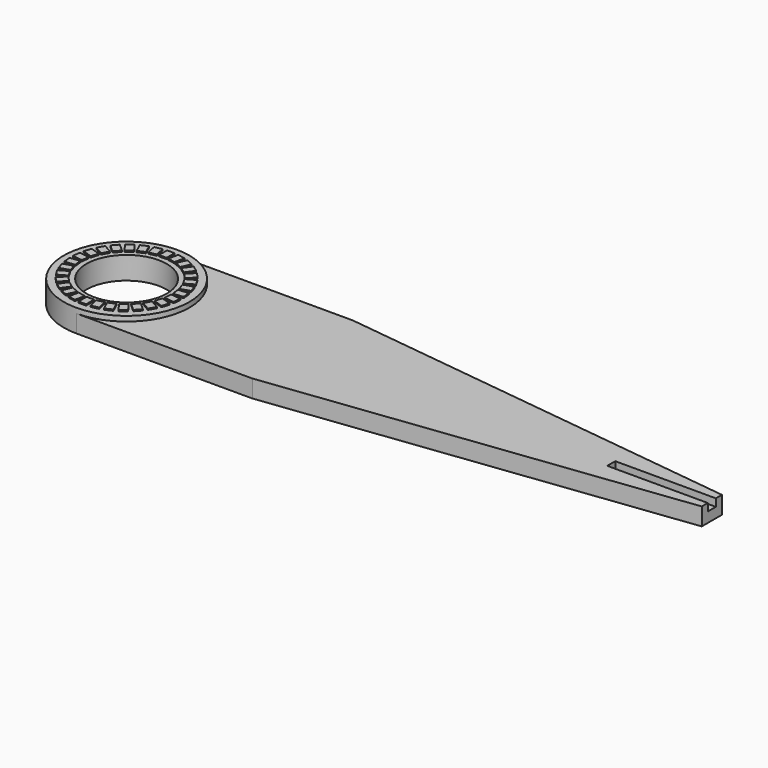
from build123d import *

# Parameters (mm, degrees)
F0_R         = 8
F1_DEPTH     = 3.5
F2_R         = 12.5
F2_R_2       = 8
F3_DEPTH     = 1
F4_W         = 1.5
F4_H         = 2
F5_DEPTH     = 0.25
F6_W         = 24.5562216001
F6_H         = 2
F6_W_2       = 20
F7_DEPTH     = 1.5
F9_TEXT_SIZE = 21.8350861027
F10_DEPTH    = 1.5


# Not quite as in the source:
# - Text() gives the source's letters only with a copy of the font that has no kerning and outlines rounded to 1/6400 em; it was checked with that copy


with BuildPart() as f1:
    # F0 (on Top) → F1 (new body)
    with BuildSketch(Plane.XY):
        with BuildLine():
            Line((35, 12.5), (0, 12.5))
            ThreePointArc((0, 12.5), (-12.5, 0), (0, -12.5))
            Line((0, -12.5), (35, -12.5))
            Line((35, -12.5), (116.3887844346, -2.5067138408))
            Line((116.3887844346, -2.5067138408), (116.3887844346, 2.5067138408))
            Line((116.3887844346, 2.5067138408), (35, 12.5))
        make_face()
        Circle(F0_R, mode=Mode.SUBTRACT)
    extrude(amount=F1_DEPTH)

    # F2 (on face) → F3 (join)
    with BuildSketch(Plane.XY.offset(3.5)):
        Circle(F2_R)
        Circle(F2_R_2, mode=Mode.SUBTRACT)
    extrude(amount=F3_DEPTH)

    # F4 (on face) → F5 (join)
    with BuildSketch(Plane.XY.offset(4.5)):
        with Locations((0, 10)):
            Rectangle(F4_W, F4_H)
        Polygon((-1.5534178984, 10.9155573762), (-3.0206392995, 10.60368984), (-2.6048159179, 8.6473946385), (-1.1375945168, 8.9592621747), align=None)
        Polygon((-3.7889439806, 10.3540525164), (-5.1592621671, 9.7439475518), (-4.3457888809, 7.9168566365), (-2.9754706945, 8.5269616011), align=None)
        Polygon((-5.8588750294, 9.3400258773), (-7.072400521, 8.4583479989), (-5.8968300164, 6.8403140102), (-4.6833045249, 7.7219918886), align=None)
        Polygon((-7.6727451255, 7.9177952891), (-8.676441035, 6.8030780508), (-7.1901513841, 5.4648168381), (-6.1864554745, 6.5795340763), align=None)
        Polygon((-9.1512794416, 6.1495190528), (-9.9012794416, 4.8504809472), (-8.1692286341, 3.8504809472), (-7.4192286341, 5.1495190528), align=None)
        Polygon((-10.2298589335, 4.1124793253), (-10.693384425, 2.6858945509), (-8.7912713924, 2.0678605622), (-8.3277459009, 3.4944453366), align=None)
        Polygon((-10.8613445016, 1.8957045175), (-11.0181371965, 0.4039216744), (-9.0290934058, 0.1948647479), (-8.8723007109, 1.6866475909), align=None)
        Polygon((-11.0181371965, -0.4039216744), (-10.8613445016, -1.8957045175), (-8.8723007109, -1.6866475909), (-9.0290934058, -0.1948647479), align=None)
        Polygon((-10.693384425, -2.6858945509), (-10.2298589335, -4.1124793253), (-8.3277459009, -3.4944453366), (-8.7912713924, -2.0678605622), align=None)
        Polygon((-9.9012794416, -4.8504809472), (-9.1512794416, -6.1495190528), (-7.4192286341, -5.1495190528), (-8.1692286341, -3.8504809472), align=None)
        Polygon((-8.676441035, -6.8030780508), (-7.6727451255, -7.9177952891), (-6.1864554745, -6.5795340763), (-7.1901513841, -5.4648168381), align=None)
        Polygon((-7.072400521, -8.4583479989), (-5.8588750294, -9.3400258773), (-4.6833045249, -7.7219918886), (-5.8968300164, -6.8403140102), align=None)
        Polygon((-5.1592621671, -9.7439475518), (-3.7889439806, -10.3540525164), (-2.9754706945, -8.5269616011), (-4.3457888809, -7.9168566365), align=None)
        Polygon((-3.0206392995, -10.60368984), (-1.5534178984, -10.9155573762), (-1.1375945168, -8.9592621747), (-2.6048159179, -8.6473946385), align=None)
        with Locations((0, -10)):
            Rectangle(F4_W, F4_H)
        Polygon((1.5534178984, -10.9155573762), (3.0206392995, -10.60368984), (2.6048159179, -8.6473946385), (1.1375945168, -8.9592621747), align=None)
        Polygon((3.7889439806, -10.3540525164), (5.1592621671, -9.7439475518), (4.3457888809, -7.9168566365), (2.9754706945, -8.5269616011), align=None)
        Polygon((5.8588750294, -9.3400258773), (7.072400521, -8.4583479989), (5.8968300164, -6.8403140102), (4.6833045249, -7.7219918886), align=None)
        Polygon((7.6727451255, -7.9177952891), (8.676441035, -6.8030780508), (7.1901513841, -5.4648168381), (6.1864554745, -6.5795340763), align=None)
        Polygon((9.1512794416, -6.1495190528), (9.9012794416, -4.8504809472), (8.1692286341, -3.8504809472), (7.4192286341, -5.1495190528), align=None)
        Polygon((10.2298589335, -4.1124793253), (10.693384425, -2.6858945509), (8.7912713924, -2.0678605622), (8.3277459009, -3.4944453366), align=None)
        Polygon((10.8613445016, -1.8957045175), (11.0181371965, -0.4039216744), (9.0290934058, -0.1948647479), (8.8723007109, -1.6866475909), align=None)
        Polygon((11.0181371965, 0.4039216744), (10.8613445016, 1.8957045175), (8.8723007109, 1.6866475909), (9.0290934058, 0.1948647479), align=None)
        Polygon((10.693384425, 2.6858945509), (10.2298589335, 4.1124793253), (8.3277459009, 3.4944453366), (8.7912713924, 2.0678605622), align=None)
        Polygon((9.9012794416, 4.8504809472), (9.1512794416, 6.1495190528), (7.4192286341, 5.1495190528), (8.1692286341, 3.8504809472), align=None)
        Polygon((8.676441035, 6.8030780508), (7.6727451255, 7.9177952891), (6.1864554745, 6.5795340763), (7.1901513841, 5.4648168381), align=None)
        Polygon((7.072400521, 8.4583479989), (5.8588750294, 9.3400258773), (4.6833045249, 7.7219918886), (5.8968300164, 6.8403140102), align=None)
        Polygon((5.1592621671, 9.7439475518), (3.7889439806, 10.3540525164), (2.9754706945, 8.5269616011), (4.3457888809, 7.9168566365), align=None)
        Polygon((3.0206392995, 10.60368984), (1.5534178984, 10.9155573762), (1.1375945168, 8.9592621747), (2.6048159179, 8.6473946385), align=None)
    extrude(amount=F5_DEPTH)

    # F6 (on face) → F7 (cut)
    with BuildSketch(Plane.XY.offset(3.5)):
        with Locations((137.6213069558, 1)):
            Rectangle(F6_W, F6_H)
        with Locations((106.3887844346, -0.0067138408)):
            Rectangle(F6_W_2, F6_H)
    extrude(amount=-F7_DEPTH, mode=Mode.SUBTRACT)

    # F9 (on line) → F10 (cut)
    with BuildSketch(Plane(origin=(0, 0, 0), x_dir=(1, 0, 0), z_dir=(0, 0, -1))):
        with Locations((15, -7.860630997)):
            Text('Max', F9_TEXT_SIZE, font='Tinos', font_style=FontStyle.ITALIC, text_align=(TextAlign.LEFT, TextAlign.BOTTOM))
    extrude(amount=-F10_DEPTH, mode=Mode.SUBTRACT)


solid = f1.part
